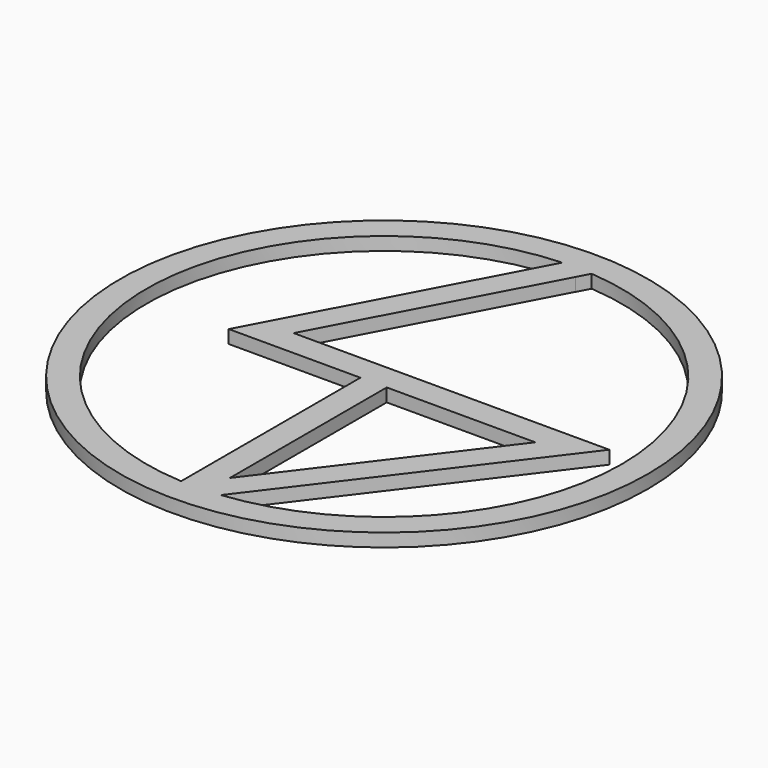
from build123d import *

# Parameters (mm, degrees)
F0_R     = 20.0378472318
F1_DEPTH = 1


with BuildPart() as f1:
    # F0 (on Top) → F1 (new body)
    with BuildSketch(Plane.XY):
        Circle(F0_R)
        with BuildLine():
            ThreePointArc((-1, -18.010106406), (-18.0377520859, 0.0585870494), (-0.8829856241, 18.0162223883))
            ThreePointArc((-0.8829856241, 18.0162223883), (0.2419860556, 18.0362239813), (1.3660161897, 17.9860482743))
            ThreePointArc((1.3660161897, 17.9860482743), (13.2288307137, 12.2622172018), (18.0378472318, 0))
            ThreePointArc((18.0378472318, 0), (13.4285198006, -12.0432050851), (1.9562398361, -17.9314544435))
            ThreePointArc((1.9562398361, -17.9314544435), (0.4797344983, -18.031466595), (-1, -18.010106406))
        make_face(mode=Mode.SUBTRACT)
        with BuildLine():
            Line((0.8829856241, 17.0774223292), (-0.8829856241, 18.0162223883))
            Line((-0.8829856241, 18.0162223883), (-10.9921143656, -1))
            Line((-10.9921143656, -1), (-1, -1))
            Line((-1, -1), (-1, -18.010106406))
            ThreePointArc((-1, -18.010106406), (0.4797344983, -18.031466595), (1.9562398361, -17.9314544435))
            Line((1.9562398361, -17.9314544435), (16.2997357547, 1))
            Line((16.2997357547, 1), (-7.6638607916, 1))
            Line((-7.6638607916, 1), (0.8829856241, 17.0774223292))
        make_face()
        Polygon((1, -15.8817395568), (1, -1), (12.2752124372, -1), align=None, mode=Mode.SUBTRACT)
        with BuildLine():
            ThreePointArc((1.3660161897, 17.9860482743), (0.2419860556, 18.0362239813), (-0.8829856241, 18.0162223883))
            Line((-0.8829856241, 18.0162223883), (0.8829856241, 17.0774223292))
            Line((0.8829856241, 17.0774223292), (1.3660161897, 17.9860482743))
        make_face()
    extrude(amount=F1_DEPTH)


solid = f1.part
